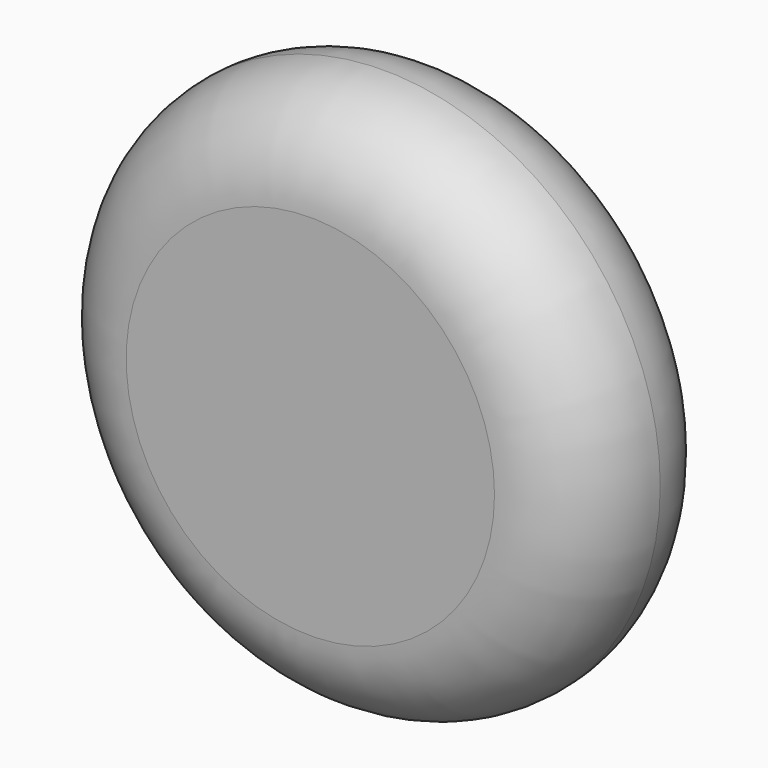
from build123d import *

# Parameters (mm, degrees)
F0_R     = 15
F1_DEPTH = 10
F2_R     = 4.99999


# Not quite as in the source:
# - a fillet or chamfer is up to 0.001 mm smaller than in the source, because OpenCascade refuses the exact size


with BuildPart() as f1:
    # F0 (on Front) → F1 (new body)
    with BuildSketch(Plane.XZ):
        Circle(F0_R)
    extrude(amount=F1_DEPTH)

    # F2 (radius 5 in the source; OpenCascade refuses exactly that, so slightly less here)
    f2_edges = [f1.edges().sort_by_distance(p)[0] for p in [
        (-15, -10, 0),
        (-15, 0, 0),
    ]]
    fillet(f2_edges, radius=F2_R)


solid = f1.part
